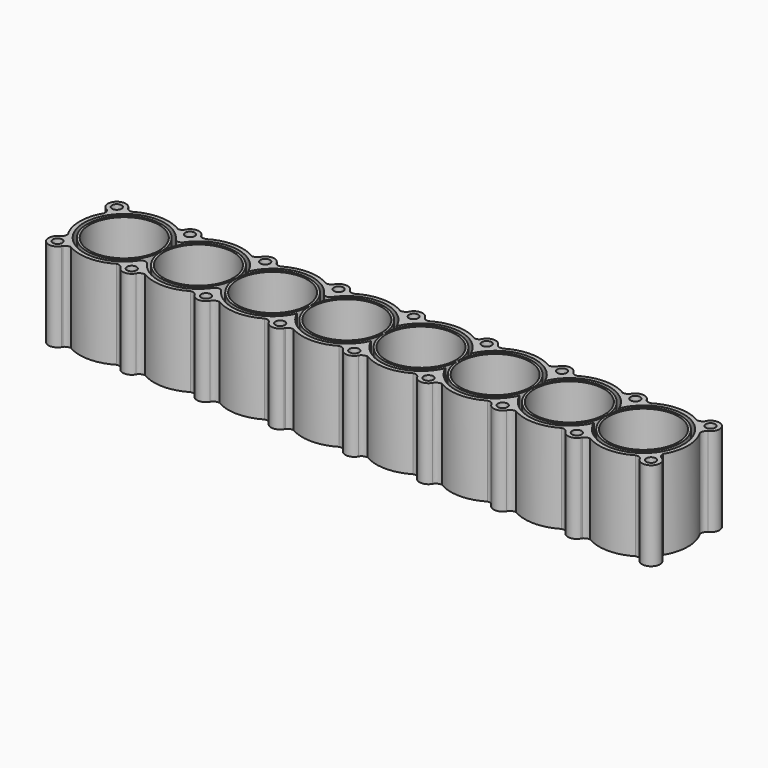
from build123d import *

# Parameters (mm, degrees)
F0_R     = 50
F0_R_2   = 47
F1_DEPTH = 120
F0_R_3   = 6.4708654687


with BuildPart() as f1:
    # F0 (on Top) → F1 (new body)
    with BuildSketch(Plane.XY):
        Circle(F0_R)
        Circle(F0_R_2, mode=Mode.SUBTRACT)
    extrude(amount=F1_DEPTH)


with BuildPart() as f1b:
    # F0 (on Top) → F1, piece 2 (new body)
    with BuildSketch(Plane.XY):
        with BuildLine():
            add(Edge.make_bspline(
                [(-51.3596856057, 31.0190698519), (-51.5025597605, 35.1747733077), (-52.9713605595, 38.468354805), (-56.1994623524, 39.5731542019)],
                knots=[0, 0, 0, 0, 9.8283161337, 9.8283161337, 9.8283161337, 9.8283161337], degree=3))
            ThreePointArc((-51.3596856057, 31.0190698519), (-59.999991062, 0.032749981), (-51.393517462, -30.9629837529))
            add(Edge.make_bspline(
                [(-55.2910167456, -39.0840672155), (-51.8487572299, -36.9356878381), (-50.8299905134, -34.2048259324), (-51.393517462, -30.9629837529)],
                knots=[0, 0, 0, 0, 8.985155217, 8.985155217, 8.985155217, 8.985155217], degree=3))
            ThreePointArc((-55.2910167456, -39.0840672155), (-58.9349957994, -58.2047728075), (-39.5736427883, -56.2002840299))
            add(Edge.make_bspline(
                [(-38.8318841421, -54.7355712372), (-39.1394115596, -55.1741066608), (-39.3892071703, -55.6613835281), (-39.5736427883, -56.2002840299)],
                knots=[8.2638945487, 8.2638945487, 8.2638945487, 8.2638945487, 9.9199315787, 9.9199315787, 9.9199315787, 9.9199315787], degree=3))
            add(Edge.make_bspline(
                [(-30.8630899122, -51.4535682054), (-34.3250387031, -51.5725908962), (-37.2972722327, -52.5472080354), (-38.8318841421, -54.7355712372)],
                knots=[0, 0, 0, 0, 8.2638945487, 8.2638945487, 8.2638945487, 8.2638945487], degree=3))
            ThreePointArc((-30.8630899122, -51.4535682054), (-0.1534728405, -59.9998037171), (30.5994627387, -51.6107825954))
            add(Edge.make_bspline(
                [(39.223346708, -55.3542727533), (37.0217623325, -51.8267650675), (33.9474805958, -50.9535160426), (30.5994627387, -51.6107825954)],
                knots=[0, 0, 0, 0, 9.4013346542, 9.4013346542, 9.4013346542, 9.4013346542], degree=3))
            ThreePointArc((39.223346708, -55.3542727533), (49.6323941008, -62.0381632645), (60.4926677825, -56.115569614))
            add(Edge.make_bspline(
                [(69.2032206586, -51.3688537895), (65.0475172028, -51.5117279443), (61.5974671793, -52.887467821), (60.4926677825, -56.115569614)],
                knots=[0, 0, 0, 0, 9.9199315787, 9.9199315787, 9.9199315787, 9.9199315787], degree=3))
            ThreePointArc((69.2032206586, -51.3688537895), (99.9128377303, -59.9150893011), (130.6657733094, -51.5260681794))
            add(Edge.make_bspline(
                [(139.2896572788, -55.2695583374), (137.0880729033, -51.7420506515), (134.0137911666, -50.8688016267), (130.6657733094, -51.5260681794)],
                knots=[0, 0, 0, 0, 9.4013346542, 9.4013346542, 9.4013346542, 9.4013346542], degree=3))
            ThreePointArc((139.2896572788, -55.2695583374), (149.6987046716, -61.9534488485), (160.5589783532, -56.030855198))
            add(Edge.make_bspline(
                [(169.2695312293, -51.2841393735), (165.1138277736, -51.4270135283), (161.6637777501, -52.8027534051), (160.5589783532, -56.030855198)],
                knots=[0, 0, 0, 0, 9.9199315787, 9.9199315787, 9.9199315787, 9.9199315787], degree=3))
            ThreePointArc((169.2695312293, -51.2841393735), (199.9791483011, -59.8303748852), (230.7320838802, -51.4413537635))
            add(Edge.make_bspline(
                [(239.3559678496, -55.1848439215), (237.1543834741, -51.6573362356), (234.0801017373, -50.7840872107), (230.7320838802, -51.4413537635)],
                knots=[0, 0, 0, 0, 9.4013346542, 9.4013346542, 9.4013346542, 9.4013346542], degree=3))
            ThreePointArc((239.3559678496, -55.1848439215), (249.7650152423, -61.8687344326), (260.625288924, -55.9461407821))
            add(Edge.make_bspline(
                [(261.3670475702, -54.4814279893), (261.0595201528, -54.919963413), (260.8097245421, -55.4072402803), (260.625288924, -55.9461407821)],
                knots=[8.2638945487, 8.2638945487, 8.2638945487, 8.2638945487, 9.9199315787, 9.9199315787, 9.9199315787, 9.9199315787], degree=3))
            add(Edge.make_bspline(
                [(269.3358418001, -51.1994249576), (265.8738930093, -51.3184476484), (262.9016594797, -52.2930647876), (261.3670475702, -54.4814279893)],
                knots=[0, 0, 0, 0, 8.2638945487, 8.2638945487, 8.2638945487, 8.2638945487], degree=3))
            ThreePointArc((269.3358418001, -51.1994249576), (300.0454588719, -59.7456604692), (330.798394451, -51.3566393475))
            add(Edge.make_bspline(
                [(339.4222784204, -55.1001295055), (337.2206940449, -51.5726218197), (334.1464123081, -50.6993727948), (330.798394451, -51.3566393475)],
                knots=[0, 0, 0, 0, 9.4013346542, 9.4013346542, 9.4013346542, 9.4013346542], degree=3))
            ThreePointArc((339.4222784204, -55.1001295055), (349.8313258131, -61.7840200166), (360.6915994948, -55.8614263662))
            add(Edge.make_bspline(
                [(369.4021523709, -51.1147105416), (365.2464489152, -51.2575846964), (361.7963988916, -52.6333245732), (360.6915994948, -55.8614263662)],
                knots=[0, 0, 0, 0, 9.9199315787, 9.9199315787, 9.9199315787, 9.9199315787], degree=3))
            ThreePointArc((369.4021523709, -51.1147105416), (400.1117694427, -59.6609460533), (430.8647050218, -51.2719249316))
            add(Edge.make_bspline(
                [(439.4885889912, -55.0154150896), (437.2870046157, -51.4879074037), (434.2127228789, -50.6146583788), (430.8647050218, -51.2719249316)],
                knots=[0, 0, 0, 0, 9.4013346542, 9.4013346542, 9.4013346542, 9.4013346542], degree=3))
            ThreePointArc((439.4885889912, -55.0154150896), (449.8976363839, -61.6993056007), (460.7579100656, -55.7767119502))
            add(Edge.make_bspline(
                [(469.4684629417, -51.0299961257), (465.312759486, -51.1728702805), (461.8627094624, -52.5486101573), (460.7579100656, -55.7767119502)],
                knots=[0, 0, 0, 0, 9.9199315787, 9.9199315787, 9.9199315787, 9.9199315787], degree=3))
            ThreePointArc((469.4684629417, -51.0299961257), (500.1780800135, -59.5762316373), (530.9310155926, -51.1872105156))
            add(Edge.make_bspline(
                [(539.5548995619, -54.9307006736), (537.3533151865, -51.4031929878), (534.2790334497, -50.5299439629), (530.9310155926, -51.1872105156)],
                knots=[0, 0, 0, 0, 9.4013346542, 9.4013346542, 9.4013346542, 9.4013346542], degree=3))
            ThreePointArc((539.5548995619, -54.9307006736), (549.9639469547, -61.6145911847), (560.8242206364, -55.6919975343))
            add(Edge.make_bspline(
                [(569.5347735125, -50.9452817097), (565.3790700568, -51.0881558645), (561.9290200332, -52.4638957413), (560.8242206364, -55.6919975343)],
                knots=[0, 0, 0, 0, 9.9199315787, 9.9199315787, 9.9199315787, 9.9199315787], degree=3))
            ThreePointArc((569.5347735125, -50.9452817097), (600.2443905842, -59.4915172214), (630.9973261634, -51.1024960997))
            add(Edge.make_bspline(
                [(639.6212101327, -54.8459862577), (637.4196257573, -51.3184785718), (634.3453440205, -50.4452295469), (630.9973261634, -51.1024960997)],
                knots=[0, 0, 0, 0, 9.4013346542, 9.4013346542, 9.4013346542, 9.4013346542], degree=3))
            ThreePointArc((639.6212101327, -54.8459862577), (650.0302575255, -61.5298767688), (660.8905312072, -55.6072831183))
            add(Edge.make_bspline(
                [(661.6322898534, -54.1425703256), (661.3247624359, -54.5811057492), (661.0749668252, -55.0683826165), (660.8905312072, -55.6072831183)],
                knots=[8.2638945487, 8.2638945487, 8.2638945487, 8.2638945487, 9.9199315787, 9.9199315787, 9.9199315787, 9.9199315787], degree=3))
            add(Edge.make_bspline(
                [(669.6010840833, -50.8605672938), (666.1391352924, -50.9795899846), (663.1669017628, -51.9542071238), (661.6322898534, -54.1425703256)],
                knots=[0, 0, 0, 0, 8.2638945487, 8.2638945487, 8.2638945487, 8.2638945487], degree=3))
            ThreePointArc((669.6010840833, -50.8605672938), (700.310701155, -59.4068028055), (731.0636367342, -51.0177816837))
            add(Edge.make_bspline(
                [(739.6875207035, -54.7612718417), (737.485936328, -51.2337641559), (734.4116545913, -50.360515131), (731.0636367342, -51.0177816837)],
                knots=[0, 0, 0, 0, 9.4013346542, 9.4013346542, 9.4013346542, 9.4013346542], degree=3))
            ThreePointArc((739.6875207035, -54.7612718417), (758.8012885356, -58.1961929692), (756.7179366343, -38.888307307))
            add(Edge.make_bspline(
                [(755.148026535, -38.1048539093), (755.6186391278, -38.4277880055), (756.141397914, -38.6909902236), (756.7179366343, -38.888307307)],
                knots=[8.0151448099, 8.0151448099, 8.0151448099, 8.0151448099, 9.7579060439, 9.7579060439, 9.7579060439, 9.7579060439], degree=3))
            add(Edge.make_bspline(
                [(751.8048595869, -30.457506379), (751.9222164292, -33.871001532), (752.9836290217, -36.6196455549), (755.148026535, -38.1048539093)],
                knots=[0, 0, 0, 0, 8.0151448099, 8.0151448099, 8.0151448099, 8.0151448099], degree=3))
            ThreePointArc((751.8048595869, -30.457506379), (760.4628644401, 0.1965858127), (752.21066478, 30.9624047828))
            add(Edge.make_bspline(
                [(756.0259360116, 39.7132180603), (752.4984283258, 37.5116336849), (751.5533982273, 34.3104226399), (752.21066478, 30.9624047828)],
                knots=[0, 0, 0, 0, 9.5463620081, 9.5463620081, 9.5463620081, 9.5463620081], degree=3))
            ThreePointArc((756.0259360116, 39.7132180603), (759.5789065269, 58.8850379905), (740.2046936304, 56.6890977459))
            add(Edge.make_bspline(
                [(739.4717209091, 55.1939109907), (739.771690956, 55.6449635805), (740.01775924, 56.1428961075), (740.2046936304, 56.6890977459)],
                knots=[8.1068477409, 8.1068477409, 8.1068477409, 8.1068477409, 9.7579060439, 9.7579060439, 9.7579060439, 9.7579060439], degree=3))
            add(Edge.make_bspline(
                [(731.7738927024, 51.7760206984), (735.2264423601, 51.8947202446), (737.998840459, 52.9792013937), (739.4717209091, 55.1939109907)],
                knots=[0, 0, 0, 0, 8.1068477409, 8.1068477409, 8.1068477409, 8.1068477409], degree=3))
            ThreePointArc((731.7738927024, 51.7760206984), (700.8625476296, 60.5916783841), (669.8368663278, 52.1872644012))
            add(Edge.make_bspline(
                [(660.9887725694, 55.0862528282), (663.1903569449, 51.5587451424), (666.4888484707, 51.5299978484), (669.8368663278, 52.1872644012)],
                knots=[0, 0, 0, 0, 9.3109020539, 9.3109020539, 9.3109020539, 9.3109020539], degree=3))
            ThreePointArc((660.9887725694, 55.0862528282), (650.9974748339, 61.8045698372), (640.1383830596, 56.6043833299))
            add(Edge.make_bspline(
                [(639.0046840614, 54.572013001), (639.4910707056, 55.1554749343), (639.8739093514, 55.8316203704), (640.1383830596, 56.6043833299)],
                knots=[7.4219981832, 7.4219981832, 7.4219981832, 7.4219981832, 9.7579060439, 9.7579060439, 9.7579060439, 9.7579060439], degree=3))
            add(Edge.make_bspline(
                [(631.7075821316, 51.6913062825), (634.8684676084, 51.799978339), (637.459263178, 52.7181498921), (639.0046840614, 54.572013001)],
                knots=[0, 0, 0, 0, 7.4219981832, 7.4219981832, 7.4219981832, 7.4219981832], degree=3))
            ThreePointArc((631.7075821316, 51.6913062825), (600.7962370588, 60.5069639682), (569.770555757, 52.1025499852))
            add(Edge.make_bspline(
                [(561.3836222174, 55.9463632732), (563.5852065929, 52.4188555874), (566.4225378999, 51.4452834325), (569.770555757, 52.1025499852)],
                knots=[0, 0, 0, 0, 9.2258091673, 9.2258091673, 9.2258091673, 9.2258091673], degree=3))
            ThreePointArc((561.3836222174, 55.9463632732), (550.8983548463, 62.5713087274), (540.0720724888, 56.519668914))
            add(Edge.make_bspline(
                [(539.3390997675, 55.0244821588), (539.6390698144, 55.4755347486), (539.8851380984, 55.9734672756), (540.0720724888, 56.519668914)],
                knots=[8.1068477409, 8.1068477409, 8.1068477409, 8.1068477409, 9.7579060439, 9.7579060439, 9.7579060439, 9.7579060439], degree=3))
            add(Edge.make_bspline(
                [(531.6412715608, 51.6065918665), (535.0938212185, 51.7252914127), (537.8662193174, 52.8097725618), (539.3390997675, 55.0244821588)],
                knots=[0, 0, 0, 0, 8.1068477409, 8.1068477409, 8.1068477409, 8.1068477409], degree=3))
            ThreePointArc((531.6412715608, 51.6065918665), (500.729926488, 60.4222495522), (469.7042451862, 52.0178355693))
            add(Edge.make_bspline(
                [(460.7309436368, 54.3872032816), (462.9325280123, 50.8596955958), (466.3562273291, 51.3605690165), (469.7042451862, 52.0178355693)],
                knots=[0, 0, 0, 0, 9.2808428525, 9.2808428525, 9.2808428525, 9.2808428525], degree=3))
            ThreePointArc((460.7309436368, 54.3872032816), (450.8579154684, 61.6685237917), (439.6806841162, 56.6124568533))
            add(Edge.make_bspline(
                [(438.3342132117, 54.1465301268), (438.9218692188, 54.9009777382), (439.3846396452, 55.7474476125), (439.6806841162, 56.6124568533)],
                knots=[7.0068196916, 7.0068196916, 7.0068196916, 7.0068196916, 9.5716637035, 9.5716637035, 9.5716637035, 9.5716637035], degree=3))
            add(Edge.make_bspline(
                [(431.57496099, 51.5218774506), (434.1913788117, 50.7111974267), (436.7288135602, 52.0854775421), (438.3342132117, 54.1465301268)],
                knots=[0, 0, 0, 0, 7.0068196916, 7.0068196916, 7.0068196916, 7.0068196916], degree=3))
            ThreePointArc((431.57496099, 51.5218774506), (400.6636159172, 60.3375351363), (369.6379346154, 51.9331211533))
            add(Edge.make_bspline(
                [(361.1374479811, 55.7191541258), (363.3390323565, 52.1916464399), (366.2899167583, 51.2758546006), (369.6379346154, 51.9331211533)],
                knots=[0, 0, 0, 0, 9.3054993788, 9.3054993788, 9.3054993788, 9.3054993788], degree=3))
            ThreePointArc((361.1374479811, 55.7191541258), (358.3861621196, 59.3501343639), (354.4895453062, 61.7102124963))
            ThreePointArc((354.4895453062, 61.7102124963), (346.2463011268, 61.6584786645), (339.9394513472, 56.3502400821))
            add(Edge.make_bspline(
                [(339.206478626, 54.8550533269), (339.5064486728, 55.3061059167), (339.7525169569, 55.8040384437), (339.9394513472, 56.3502400821)],
                knots=[8.1068477409, 8.1068477409, 8.1068477409, 8.1068477409, 9.7579060439, 9.7579060439, 9.7579060439, 9.7579060439], degree=3))
            add(Edge.make_bspline(
                [(331.5086504192, 51.4371630347), (334.9612000769, 51.5558625808), (337.7335981758, 52.6403437299), (339.206478626, 54.8550533269)],
                knots=[0, 0, 0, 0, 8.1068477409, 8.1068477409, 8.1068477409, 8.1068477409], degree=3))
            ThreePointArc((331.5086504192, 51.4371630347), (300.5973053465, 60.2528207203), (269.5716240447, 51.8484067374))
            add(Edge.make_bspline(
                [(260.7235302862, 54.7473951645), (262.9251146617, 51.2198874786), (266.2236061876, 51.1911401846), (269.5716240447, 51.8484067374)],
                knots=[0, 0, 0, 0, 9.3109020539, 9.3109020539, 9.3109020539, 9.3109020539], degree=3))
            ThreePointArc((260.7235302862, 54.7473951645), (250.7322325507, 61.4657121734), (239.8731407764, 56.2655256661))
            add(Edge.make_bspline(
                [(238.7394417783, 54.2331553372), (239.2258284224, 54.8166172705), (239.6086670682, 55.4927627066), (239.8731407764, 56.2655256661)],
                knots=[7.4219981832, 7.4219981832, 7.4219981832, 7.4219981832, 9.7579060439, 9.7579060439, 9.7579060439, 9.7579060439], degree=3))
            add(Edge.make_bspline(
                [(231.4423398484, 51.3524486187), (234.6032253253, 51.4611206753), (237.1940208949, 52.3792922283), (238.7394417783, 54.2331553372)],
                knots=[0, 0, 0, 0, 7.4219981832, 7.4219981832, 7.4219981832, 7.4219981832], degree=3))
            ThreePointArc((231.4423398484, 51.3524486187), (200.5309947757, 60.1681063044), (169.5053134739, 51.7636923214))
            add(Edge.make_bspline(
                [(161.1183799343, 55.6075056094), (163.3199643097, 52.0799979236), (166.1572956168, 51.1064257687), (169.5053134739, 51.7636923214)],
                knots=[0, 0, 0, 0, 9.2258091673, 9.2258091673, 9.2258091673, 9.2258091673], degree=3))
            ThreePointArc((161.1183799343, 55.6075056094), (150.6331125631, 62.2324510636), (139.8068302056, 56.1808112502))
            add(Edge.make_bspline(
                [(139.0738574844, 54.685624495), (139.3738275312, 55.1366770848), (139.6198958153, 55.6346096118), (139.8068302056, 56.1808112502)],
                knots=[8.1068477409, 8.1068477409, 8.1068477409, 8.1068477409, 9.7579060439, 9.7579060439, 9.7579060439, 9.7579060439], degree=3))
            add(Edge.make_bspline(
                [(131.3760292776, 51.2677342028), (134.8285789353, 51.3864337489), (137.6009770342, 52.470914898), (139.0738574844, 54.685624495)],
                knots=[0, 0, 0, 0, 8.1068477409, 8.1068477409, 8.1068477409, 8.1068477409], degree=3))
            ThreePointArc((131.3760292776, 51.2677342028), (100.4646842049, 60.0833918884), (69.4390029031, 51.6789779055))
            add(Edge.make_bspline(
                [(60.4657013537, 54.0483456178), (62.6672857292, 50.520837932), (66.090985046, 51.0217113527), (69.4390029031, 51.6789779055)],
                knots=[0, 0, 0, 0, 9.2808428525, 9.2808428525, 9.2808428525, 9.2808428525], degree=3))
            ThreePointArc((60.4657013537, 54.0483456178), (50.5926731852, 61.329666128), (39.415441833, 56.2735991895))
            add(Edge.make_bspline(
                [(38.0689709285, 53.807672463), (38.6566269357, 54.5621200744), (39.1193973621, 55.4085899487), (39.415441833, 56.2735991895)],
                knots=[7.0068196916, 7.0068196916, 7.0068196916, 7.0068196916, 9.5716637035, 9.5716637035, 9.5716637035, 9.5716637035], degree=3))
            add(Edge.make_bspline(
                [(31.3097187068, 51.1830197868), (33.9261365285, 50.372339763), (36.4635712771, 51.7466198784), (38.0689709285, 53.807672463)],
                knots=[0, 0, 0, 0, 7.0068196916, 7.0068196916, 7.0068196916, 7.0068196916], degree=3))
            ThreePointArc((31.3097187068, 51.1830197868), (0.3983736341, 59.9986774725), (-30.6273076677, 51.5942634895))
            add(Edge.make_bspline(
                [(-39.1277943021, 55.380296462), (-36.9262099266, 51.8527887762), (-33.9753255248, 50.9369969368), (-30.6273076677, 51.5942634895)],
                knots=[0, 0, 0, 0, 9.3054993788, 9.3054993788, 9.3054993788, 9.3054993788], degree=3))
            ThreePointArc((-39.1277943021, 55.380296462), (-58.2416666519, 58.9009762136), (-56.1994623524, 39.5731542019))
        make_face()
        with Locations((-50, -50)):
            Circle(F0_R_3, mode=Mode.SUBTRACT)
        with Locations((50.0663105708, -49.9152855841)):
            Circle(F0_R_3, mode=Mode.SUBTRACT)
        with Locations((150.1326211416, -49.8305711681)):
            Circle(F0_R_3, mode=Mode.SUBTRACT)
        with Locations((250.1989317124, -49.7458567522)):
            Circle(F0_R_3, mode=Mode.SUBTRACT)
        with Locations((350.2652422831, -49.6611423362)):
            Circle(F0_R_3, mode=Mode.SUBTRACT)
        with BuildLine():
            ThreePointArc((44.8328308062, -30.8797245781), (-54.4383870458, -0.0460866013), (44.7804820937, 30.9555896662))
            ThreePointArc((44.7804820937, 30.9555896662), (50.0093036047, 28.216424933), (55.2334797645, 30.9644389941))
            ThreePointArc((55.2334797645, 30.9644389941), (105.4264755312, 54.2585894824), (150.0813043101, 21.5798419889))
            ThreePointArc((150.0813043101, 21.5798419889), (194.68073859, 54.3341506051), (244.9131032352, 31.1250184981))
            ThreePointArc((244.9131032352, 31.1250184981), (250.1419247462, 28.3858537649), (255.3661009061, 31.133867826))
            ThreePointArc((255.3661009061, 31.133867826), (305.5590966728, 54.4280183143), (350.2139254517, 21.7492708208))
            ThreePointArc((350.2139254517, 21.7492708208), (400.2191556818, 54.7772447096), (450.2802360224, 21.8339852368))
            ThreePointArc((450.2802360224, 21.8339852368), (500.2854662526, 54.8619591255), (550.3465465932, 21.9186996527))
            ThreePointArc((550.3465465932, 21.9186996527), (600.3517768234, 54.9466735415), (650.412857164, 22.0034140687))
            ThreePointArc((650.412857164, 22.0034140687), (754.9025610413, 0.639087513), (650.4491802562, -20.9021266614))
            ThreePointArc((650.4491802562, -20.9021266614), (600.4439500261, -53.9301005501), (550.3828696854, -20.9868410773))
            ThreePointArc((550.3828696854, -20.9868410773), (500.3776394553, -54.0148149661), (450.3165591146, -21.0715554933))
            ThreePointArc((450.3165591146, -21.0715554933), (400.3113288845, -54.099529382), (350.2502485438, -21.1562699092))
            ThreePointArc((350.2502485438, -21.1562699092), (300.2450183137, -54.1842437979), (250.1839379731, -21.2409843252))
            ThreePointArc((250.1839379731, -21.2409843252), (205.5845036931, -53.9952929413), (155.3521390479, -30.7861608343))
            ThreePointArc((155.3521390479, -30.7861608343), (150.1233175369, -28.0469961012), (144.899141377, -30.7950101622))
            ThreePointArc((144.899141377, -30.7950101622), (100.1123971721, -54.3536726298), (55.2858284771, -30.8708752502))
            ThreePointArc((55.2858284771, -30.8708752502), (50.0570069661, -28.1317105171), (44.8328308062, -30.8797245781))
        make_face(mode=Mode.SUBTRACT)
        with Locations((450.3315528539, -49.5764279203)):
            Circle(F0_R_3, mode=Mode.SUBTRACT)
        with Locations((550.3978634247, -49.4917135043)):
            Circle(F0_R_3, mode=Mode.SUBTRACT)
        with Locations((650.4641739955, -49.4069990884)):
            Circle(F0_R_3, mode=Mode.SUBTRACT)
        with Locations((750.5304845663, -49.3222846724)):
            Circle(F0_R_3, mode=Mode.SUBTRACT)
        with Locations((-50, 50)):
            Circle(F0_R_3, mode=Mode.SUBTRACT)
        with Locations((49.3174310516, 49.2662418936)):
            Circle(F0_R_3, mode=Mode.SUBTRACT)
        with Locations((150.1326211416, 50.1694288319)):
            Circle(F0_R_3, mode=Mode.SUBTRACT)
        with Locations((249.8513245883, 49.3670987025)):
            Circle(F0_R_3, mode=Mode.SUBTRACT)
        with BuildLine():
            ThreePointArc((348.1456521544, 44.2249851103), (344.3566423556, 52.482583095), (352.5591134054, 56.3894985545))
            ThreePointArc((352.5591134054, 56.3894985545), (356.3481232042, 48.1319005698), (348.1456521544, 44.2249851103))
        make_face(mode=Mode.SUBTRACT)
        with Locations((449.5826733348, 49.6050995574)):
            Circle(F0_R_3, mode=Mode.SUBTRACT)
        with Locations((550.3978634247, 50.5082864957)):
            Circle(F0_R_3, mode=Mode.SUBTRACT)
        with Locations((650.1165668715, 49.7059563662)):
            Circle(F0_R_3, mode=Mode.SUBTRACT)
        with Locations((750.7047655598, 50.6144836648)):
            Circle(F0_R_3, mode=Mode.SUBTRACT)
        with BuildLine():
            ThreePointArc((39.415441833, 56.2735991895), (38.6705735108, 55.0797495493), (38.0689709285, 53.807672463))
            add(Edge.make_bspline(
                [(38.0689709285, 53.807672463), (38.6566269357, 54.5621200744), (39.1193973621, 55.4085899487), (39.415441833, 56.2735991895)],
                knots=[7.0068196916, 7.0068196916, 7.0068196916, 7.0068196916, 9.5716637035, 9.5716637035, 9.5716637035, 9.5716637035], degree=3))
        make_face()
        with BuildLine():
            ThreePointArc((139.8068302056, 56.1808112502), (139.4146578792, 55.4458096857), (139.0738574844, 54.685624495))
            add(Edge.make_bspline(
                [(139.0738574844, 54.685624495), (139.3738275312, 55.1366770848), (139.6198958153, 55.6346096118), (139.8068302056, 56.1808112502)],
                knots=[8.1068477409, 8.1068477409, 8.1068477409, 8.1068477409, 9.7579060439, 9.7579060439, 9.7579060439, 9.7579060439], degree=3))
        make_face()
        with BuildLine():
            ThreePointArc((239.8731407764, 56.2655256661), (239.2574414561, 55.2765899614), (238.7394417783, 54.2331553372))
            add(Edge.make_bspline(
                [(238.7394417783, 54.2331553372), (239.2258284224, 54.8166172705), (239.6086670682, 55.4927627066), (239.8731407764, 56.2655256661)],
                knots=[7.4219981832, 7.4219981832, 7.4219981832, 7.4219981832, 9.7579060439, 9.7579060439, 9.7579060439, 9.7579060439], degree=3))
        make_face()
        with BuildLine():
            ThreePointArc((339.9394513472, 56.3502400821), (339.5472790208, 55.6152385176), (339.206478626, 54.8550533269))
            add(Edge.make_bspline(
                [(339.206478626, 54.8550533269), (339.5064486728, 55.3061059167), (339.7525169569, 55.8040384437), (339.9394513472, 56.3502400821)],
                knots=[8.1068477409, 8.1068477409, 8.1068477409, 8.1068477409, 9.7579060439, 9.7579060439, 9.7579060439, 9.7579060439], degree=3))
        make_face()
        with BuildLine():
            ThreePointArc((439.6806841162, 56.6124568533), (438.935815794, 55.4186072131), (438.3342132117, 54.1465301268))
            add(Edge.make_bspline(
                [(438.3342132117, 54.1465301268), (438.9218692188, 54.9009777382), (439.3846396452, 55.7474476125), (439.6806841162, 56.6124568533)],
                knots=[7.0068196916, 7.0068196916, 7.0068196916, 7.0068196916, 9.5716637035, 9.5716637035, 9.5716637035, 9.5716637035], degree=3))
        make_face()
        with BuildLine():
            ThreePointArc((540.0720724888, 56.519668914), (539.6799001623, 55.7846673495), (539.3390997675, 55.0244821588))
            add(Edge.make_bspline(
                [(539.3390997675, 55.0244821588), (539.6390698144, 55.4755347486), (539.8851380984, 55.9734672756), (540.0720724888, 56.519668914)],
                knots=[8.1068477409, 8.1068477409, 8.1068477409, 8.1068477409, 9.7579060439, 9.7579060439, 9.7579060439, 9.7579060439], degree=3))
        make_face()
        with BuildLine():
            ThreePointArc((640.1383830596, 56.6043833299), (639.5226837393, 55.6154476251), (639.0046840614, 54.572013001))
            add(Edge.make_bspline(
                [(639.0046840614, 54.572013001), (639.4910707056, 55.1554749343), (639.8739093514, 55.8316203704), (640.1383830596, 56.6043833299)],
                knots=[7.4219981832, 7.4219981832, 7.4219981832, 7.4219981832, 9.7579060439, 9.7579060439, 9.7579060439, 9.7579060439], degree=3))
        make_face()
        with BuildLine():
            add(Edge.make_bspline(
                [(755.148026535, -38.1048539093), (755.6186391278, -38.4277880055), (756.141397914, -38.6909902236), (756.7179366343, -38.888307307)],
                knots=[8.0151448099, 8.0151448099, 8.0151448099, 8.0151448099, 9.7579060439, 9.7579060439, 9.7579060439, 9.7579060439], degree=3))
            ThreePointArc((756.7179366343, -38.888307307), (755.9471647156, -38.4681599764), (755.148026535, -38.1048539093))
        make_face()
        with BuildLine():
            ThreePointArc((740.2046936304, 56.6890977459), (739.8125213039, 55.9540961814), (739.4717209091, 55.1939109907))
            add(Edge.make_bspline(
                [(739.4717209091, 55.1939109907), (739.771690956, 55.6449635805), (740.01775924, 56.1428961075), (740.2046936304, 56.6890977459)],
                knots=[8.1068477409, 8.1068477409, 8.1068477409, 8.1068477409, 9.7579060439, 9.7579060439, 9.7579060439, 9.7579060439], degree=3))
        make_face()
    extrude(amount=F1_DEPTH)


with BuildPart() as f1c:
    # F0 (on Top) → F1, piece 3 (new body)
    with BuildSketch(Plane.XY):
        with Locations((100.0663105708, 0.0847144159)):
            Circle(F0_R)
        with Locations((100.0663105708, 0.0847144159)):
            Circle(F0_R_2, mode=Mode.SUBTRACT)
    extrude(amount=F1_DEPTH)


with BuildPart() as f1d:
    # F0 (on Top) → F1, piece 4 (new body)
    with BuildSketch(Plane.XY):
        with Locations((200.1326211416, 0.1694288319)):
            Circle(F0_R)
        with Locations((200.1326211416, 0.1694288319)):
            Circle(F0_R_2, mode=Mode.SUBTRACT)
    extrude(amount=F1_DEPTH)


with BuildPart() as f1e:
    # F0 (on Top) → F1, piece 5 (new body)
    with BuildSketch(Plane.XY):
        with Locations((300.1989317124, 0.2541432478)):
            Circle(F0_R)
        with Locations((300.1989317124, 0.2541432478)):
            Circle(F0_R_2, mode=Mode.SUBTRACT)
    extrude(amount=F1_DEPTH)


with BuildPart() as f1f:
    # F0 (on Top) → F1, piece 6 (new body)
    with BuildSketch(Plane.XY):
        with Locations((400.2652422831, 0.3388576638)):
            Circle(F0_R)
        with Locations((400.2652422831, 0.3388576638)):
            Circle(F0_R_2, mode=Mode.SUBTRACT)
    extrude(amount=F1_DEPTH)


with BuildPart() as f1g:
    # F0 (on Top) → F1, piece 7 (new body)
    with BuildSketch(Plane.XY):
        with Locations((500.3315528539, 0.4235720797)):
            Circle(F0_R)
        with Locations((500.3315528539, 0.4235720797)):
            Circle(F0_R_2, mode=Mode.SUBTRACT)
    extrude(amount=F1_DEPTH)


with BuildPart() as f1h:
    # F0 (on Top) → F1, piece 8 (new body)
    with BuildSketch(Plane.XY):
        with Locations((600.3978634247, 0.5082864957)):
            Circle(F0_R)
        with Locations((600.3978634247, 0.5082864957)):
            Circle(F0_R_2, mode=Mode.SUBTRACT)
    extrude(amount=F1_DEPTH)


with BuildPart() as f1i:
    # F0 (on Top) → F1, piece 9 (new body)
    with BuildSketch(Plane.XY):
        with Locations((700.4641739955, 0.5930009116)):
            Circle(F0_R)
        with Locations((700.4641739955, 0.5930009116)):
            Circle(F0_R_2, mode=Mode.SUBTRACT)
    extrude(amount=F1_DEPTH)


solid = Compound([f1.part, f1b.part, f1c.part, f1d.part, f1e.part, f1f.part, f1g.part, f1h.part, f1i.part])
